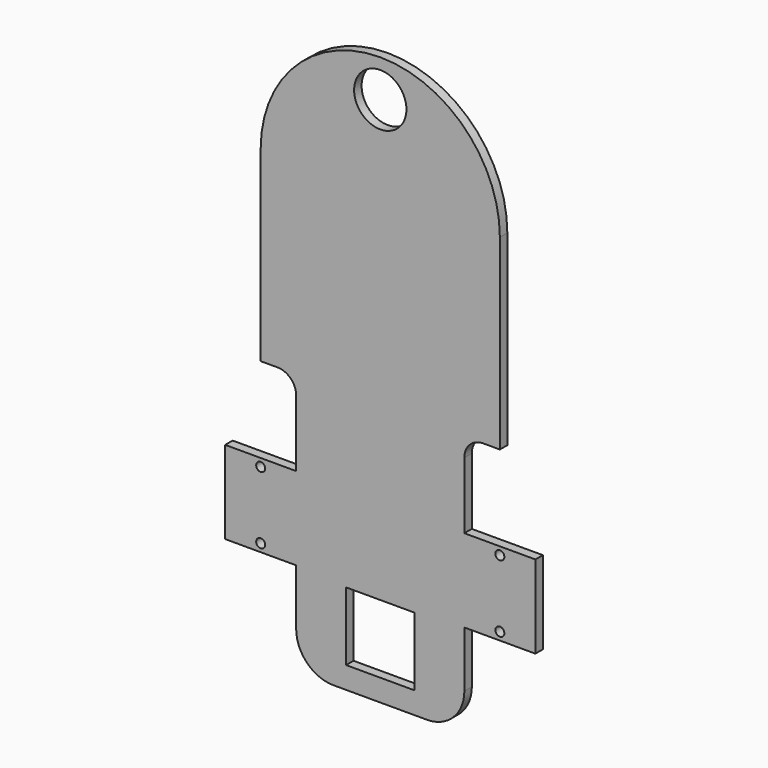
from build123d import *

# Parameters (mm, degrees)
F0_R     = 1.524
F0_W     = 23.241
F0_H     = 23.241
F0_R_2   = 8.89
F1_DEPTH = 1.5875


# Not quite as in the source:
# - a length typed as a fraction of an inch, garbled in the dataset ("3 / 203.2 mm" for 3/8 in), is restored


with BuildPart() as f1:
    # F0 (on Front) → F1 (new body, symmetric)
    with BuildSketch(Plane.XZ):
        with BuildLine():
            Line((34.925, -31.75), (40.6399987437, -31.75))
            Line((40.6399987437, -31.75), (40.6400012563, 31.75))
            ThreePointArc((40.6400012563, 31.75), (1.2563e-06, 72.3900018664), (-40.6399987437, 31.75))
            Line((-40.6399987437, 31.75), (-40.6400012563, -31.75))
            Line((-40.6400012563, -31.75), (-34.925, -31.75))
            ThreePointArc((-34.925, -31.75), (-30.4348719395, -33.6098719395), (-28.575, -38.1))
            Line((-28.575, -38.1), (-28.575, -60.706))
            Line((-28.575, -60.706), (-52.705, -60.706))
            Line((-52.705, -60.706), (-52.705, -88.9))
            Line((-52.705, -88.9), (-28.575, -88.9))
            Line((-28.575, -88.9), (-28.575, -107.95))
            ThreePointArc((-28.575, -107.95), (-24.8552561211, -116.9302561211), (-15.875, -120.65))
            Line((-15.875, -120.65), (15.875, -120.65))
            ThreePointArc((15.875, -120.65), (24.8552561211, -116.9302561211), (28.575, -107.95))
            Line((28.575, -107.95), (28.575, -88.9))
            Line((28.575, -88.9), (52.705, -88.9))
            Line((52.705, -88.9), (52.705, -60.706))
            Line((52.705, -60.706), (28.575, -60.706))
            Line((28.575, -60.706), (28.575, -38.1))
            ThreePointArc((28.575, -38.1), (30.4348719395, -33.6098719395), (34.925, -31.75))
        make_face()
        with Locations((-40.64, -86.233)):
            Circle(F0_R, mode=Mode.SUBTRACT)
        with Locations((-40.64, -63.373)):
            Circle(F0_R, mode=Mode.SUBTRACT)
        with Locations((0, -101.6)):
            Rectangle(F0_W, F0_H, mode=Mode.SUBTRACT)
        with Locations((40.64, -86.233)):
            Circle(F0_R, mode=Mode.SUBTRACT)
        with Locations((40.64, -63.373)):
            Circle(F0_R, mode=Mode.SUBTRACT)
        with Locations((0, 59.6900018664)):
            Circle(F0_R_2, mode=Mode.SUBTRACT)
    extrude(amount=F1_DEPTH, both=True)


solid = f1.part
